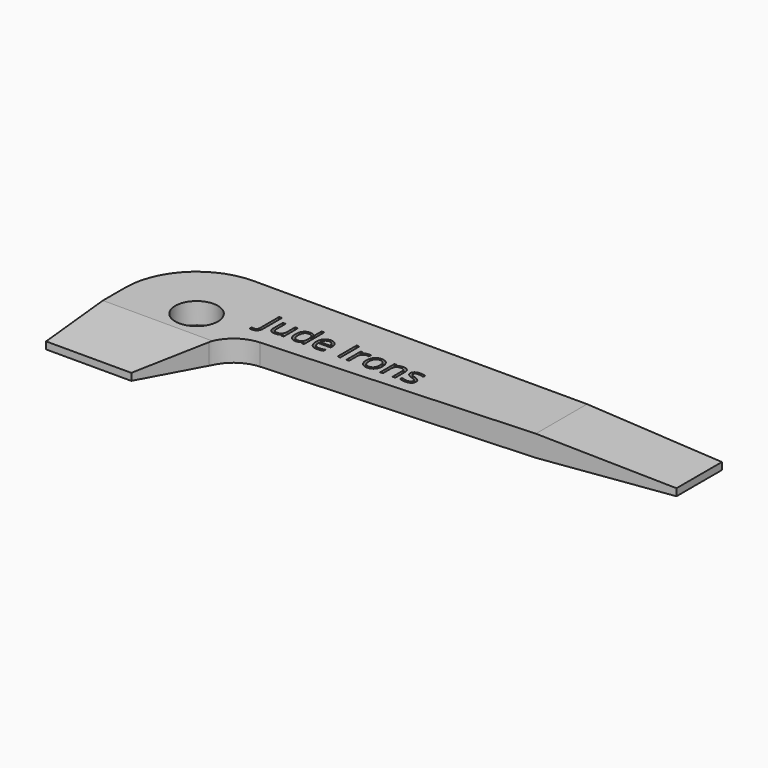
from build123d import *

# Parameters (mm, degrees)
F0_R         = 2.38125
F1_DEPTH     = 2.38125
F3_DEPTH     = 25.4
F5_DEPTH     = 25.4
F6_TEXT_SIZE = 3.7298744751
F7_DEPTH     = 0.508


# Not quite as in the source:
# - Text() gives the source's letters only with a copy of the font that has no kerning and outlines rounded to 1/6400 em; it was checked with that copy


with BuildPart() as f1:
    # F0 (on Top) → F1 (new body)
    with BuildSketch(Plane.XY):
        with BuildLine():
            Line((0, 11.1125), (0, 0))
            Line((0, 0), (9.525, 0))
            Line((9.525, 0), (12.1173647876, 7.6271664624))
            ThreePointArc((12.1173647876, 7.6271664624), (13.4786145605, 9.5135918491), (15.6631963617, 10.3130942181))
            Line((15.6631963617, 10.3130942181), (60.325, 12.7))
            Line((60.325, 12.7), (60.325, 19.05))
            Line((60.325, 19.05), (7.9375, 19.05))
            ThreePointArc((7.9375, 19.05), (2.3248399243, 16.7251600757), (0, 11.1125))
        make_face()
        with Locations((7.9375, 11.1125)):
            Circle(F0_R, mode=Mode.SUBTRACT)
    extrude(amount=F1_DEPTH)

    # F2 (on face) → F3 (cut)
    with BuildSketch(Plane(origin=(0, 19.05, 0), x_dir=(-1, 0, 0), z_dir=(0, 1, 0))):
        Polygon((-60.325, 1.5875), (-45.24375, 2.38125), (-60.325, 2.38125), align=None)
        Polygon((-60.325, 0), (-45.24375, 0), (-60.325, 0.79375), align=None)
    extrude(amount=-F3_DEPTH, mode=Mode.SUBTRACT)

    # F4 (on face) → F5 (cut)
    with BuildSketch(Plane(origin=(0, 0, 0), x_dir=(0, -1, 0), z_dir=(-1, 0, 0))):
        Polygon((0, 2.38125), (-7.9375, 2.38125), (0, 1.5875), align=None)
        Polygon((0, 0.79375), (-7.9375, 0), (0, 0), align=None)
    extrude(amount=-F5_DEPTH, mode=Mode.SUBTRACT)

    # F6 (on face) → F7 (cut)
    with BuildSketch(Plane.XY.offset(2.38125)):
        with Locations((13.6108500883, 12.4746952206)):
            Text('Jude Irons', F6_TEXT_SIZE, font='Open Sans', text_align=(TextAlign.LEFT, TextAlign.BOTTOM))
    extrude(amount=-F7_DEPTH, mode=Mode.SUBTRACT)


solid = f1.part
